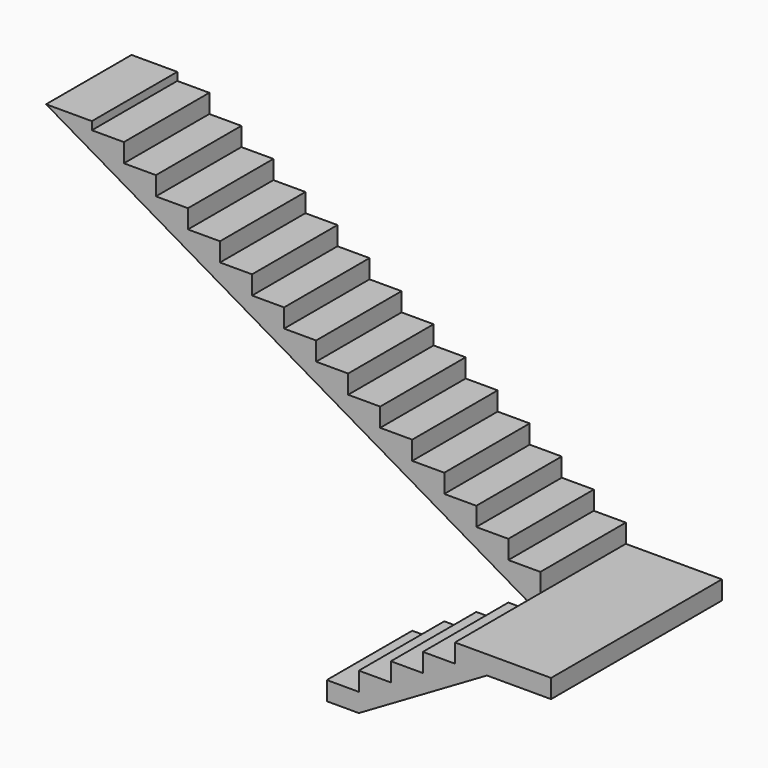
from build123d import *

# Parameters (mm, degrees)
F0_W     = 9144
F0_H     = 2032
F1_DEPTH = 3454.4
F3_DEPTH = 1016
F5_DEPTH = 1016


# Not quite as in the source:
# - a feature names something its author has since deleted; it is built from what else it names


with BuildPart() as f1:
    # F0 (on Top) → F1 (new body)
    with BuildSketch(Plane.XY):
        with Locations((-4572, -1016)):
            Rectangle(F0_W, F0_H)
    extrude(amount=F1_DEPTH)

    # F2 (on face) → F3 (cut)
    with BuildSketch(Plane.XZ.offset(2032)):
        Polygon((-2341.2702168835, 0), (-2133.6, 0), (-2133.6, 177.8), (-1828.8, 177.8), (-1828.8, 355.6), (-1524, 355.6), (-1524, 533.4), (-1219.2, 533.4), (-1219.2, 711.2), (-914.4, 711.2), (-914.4, 889), (0, 889), (0, 3454.4), (-9144, 3454.4), (-9144, 0), align=None)
        Polygon((-609.6, 711.2), (-1828.8, 0), (0, 0), (0, 711.2), align=None)
    extrude(amount=-F3_DEPTH, mode=Mode.SUBTRACT)

    # F4 (on face) → F5 (cut, through all)
    with BuildSketch(Plane.XZ.offset(1016)):
        Polygon((-1219.2, 711.2), (-914.4, 711.2), (-5617.0285714286, 3454.4), (-9144, 3454.4), (-9144, 0), (-2133.6, 0), (-2133.6, 177.8), (-1828.8, 177.8), (-1828.8, 355.6), (-1524, 355.6), (-1524, 533.4), (-1219.2, 533.4), align=None)
        Polygon((-914.4, 1066.8), (-914.4, 889), (0, 889), (0, 3454.4), (-5181.6, 3454.4), (-5181.6, 3378.2), (-4876.8, 3378.2), (-4876.8, 3200.4), (-4572, 3200.4), (-4572, 3022.6), (-4267.2, 3022.6), (-4267.2, 2844.8), (-3962.4, 2844.8), (-3962.4, 2667), (-3657.6, 2667), (-3657.6, 2489.2), (-3352.8, 2489.2), (-3352.8, 2311.4), (-3048, 2311.4), (-3048, 2133.6), (-2743.2, 2133.6), (-2743.2, 1955.8), (-2438.4, 1955.8), (-2438.4, 1778), (-2133.6, 1778), (-2133.6, 1600.2), (-1828.8, 1600.2), (-1828.8, 1422.4), (-1524, 1422.4), (-1524, 1244.6), (-1219.2, 1244.6), (-1219.2, 1066.8), align=None)
        Polygon((0, 711.2), (-914.4, 711.2), (-1219.2, 711.2), (-1219.2, 533.4), (-1524, 533.4), (-1524, 355.6), (-1828.8, 355.6), (-1828.8, 177.8), (-2133.6, 177.8), (-2133.6, 0), (0, 0), align=None)
    extrude(amount=-F5_DEPTH, mode=Mode.SUBTRACT)


solid = f1.part
